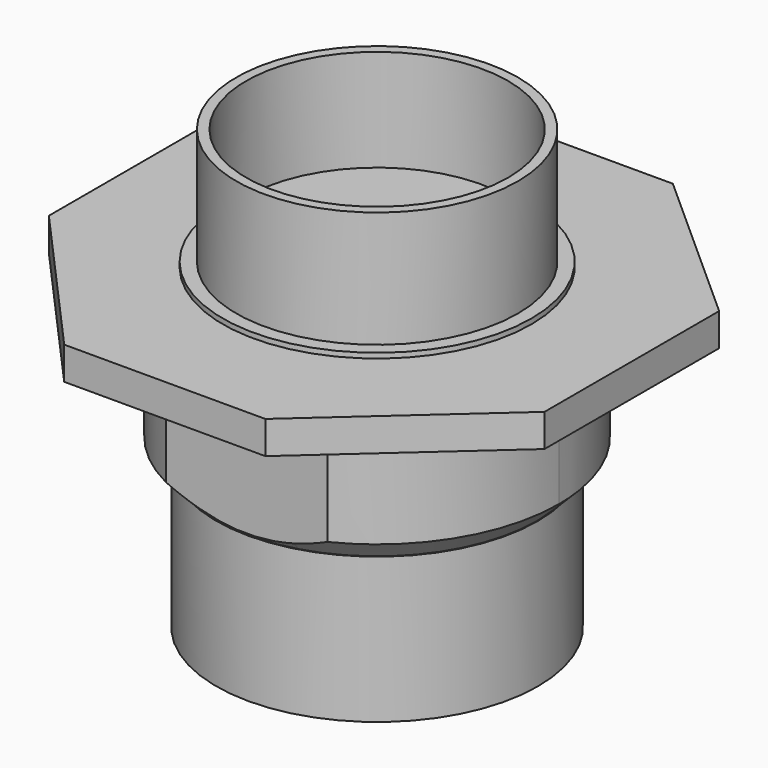
from build123d import *

# Parameters (mm, degrees)
F1_DEPTH    = 2.25
F2_R        = 10.6
F3_DEPTH    = 10.6
F5_DEPTH    = 9.5
F6_T2_ANGLE = 286.1981288485
F6_T4_ANGLE = 106.0815039342
F7_R        = 11.05
F8_DEPTH    = 10
F9_R        = 9
F10_DEPTH   = 7
F11_R       = 10.6
F11_R_2     = 9.6734059383
F12_DEPTH   = 8
F13_R       = 9.375
F14_DEPTH   = 1


# Not quite as in the source:
# - a fillet or chamfer that OpenCascade refuses, or shapes differently, is made with other operations: its cross-section is extruded or revolved along the edge and cut away or added


with BuildPart() as f1:
    # F0 (on Top) → F1 (new body)
    with BuildSketch(Plane.XY):
        Polygon((0, 11.1803398875), (10, 0), (23.8196601125, 0), (35, 10), (35, 25), (23.8196601125, 35), (10, 35), (0, 23.8196601125), align=None)
    extrude(amount=F1_DEPTH)

    # F2 (on Top) → F3 (join)
    with BuildSketch(Plane.XY):
        with Locations((17.5, 17.5)):
            Circle(F2_R)
    extrude(amount=F3_DEPTH)

    # F4 (on face) → F5 (join)
    with BuildSketch(Plane(origin=(0, 0, 0), x_dir=(1, 0, 0), z_dir=(0, 0, -1))):
        with BuildLine():
            ThreePointArc((11.9493243654, -6.3), (10.909607198, -28.1215216761), (30, -17.5))
            ThreePointArc((30, -17.5), (28.1215216761, -10.909607198), (23.0506756346, -6.3))
            Line((23.0506756346, -6.3), (11.9493243654, -6.3))
        make_face()
    extrude(amount=F5_DEPTH)

    # F6: chamfer of 1.5 on 2 edges, made by hand

    # F6_s1 → F6_t2 (revolve, cut)
    with BuildSketch(Plane(origin=(20.8261774668, 6.0498263405, 0), x_dir=(0, 0, 1), z_dir=(0.9603027964, 0.2789597449, 0))):
        with BuildLine():
            Line((-7.9575735931, 0.618923005), (-9.5424264069, -0.9659298087))
            Line((-9.5424264069, -0.9659298087), (-9.5724264069, -0.9659298087))
            ThreePointArc((-9.5724264069, -0.9659298087), (-9.53, -0.1947166053), (-9.53, 0.5764965982))
            Line((-9.53, 0.5764965982), (-9.5, 0.6064965982))
            ThreePointArc((-9.5, 0.6064965982), (-8.7287867966, 0.6064965982), (-7.9575735931, 0.648923005))
            Line((-7.9575735931, 0.648923005), (-7.9575735931, 0.618923005))
        make_face()
    revolve(axis=Axis((17.5, 17.5, -9.5), (0, 0, -1)), revolution_arc=F6_T2_ANGLE, mode=Mode.SUBTRACT)

    # F6_s3 → F6_t4 (revolve, cut)
    with BuildSketch(Plane.XZ.offset(-17.5)):
        with BuildLine():
            Line((30.0424264069, -7.9575735931), (28.4575735931, -9.5424264069))
            Line((28.4575735931, -9.5424264069), (28.4575735931, -9.5724264069))
            ThreePointArc((28.4575735931, -9.5724264069), (29.2287867966, -9.53), (30, -9.53))
            Line((30, -9.53), (30.03, -9.5))
            ThreePointArc((30.03, -9.5), (30.03, -8.7287867966), (30.0724264069, -7.9575735931))
            Line((30.0724264069, -7.9575735931), (30.0424264069, -7.9575735931))
        make_face()
    revolve(axis=Axis((17.5, 17.5, -9.5), (0, 0, -1)), revolution_arc=F6_T4_ANGLE, mode=Mode.SUBTRACT)

    # F7 (on face) → F8 (join)
    with BuildSketch(Plane(origin=(0, 0, -9.5), x_dir=(1, 0, 0), z_dir=(0, 0, -1))):
        with Locations((17.5, -17.5)):
            Circle(F7_R)
    extrude(amount=F8_DEPTH)

    # F9 (on face) → F10 (cut)
    with BuildSketch(Plane.XY.offset(10.6)):
        with Locations((17.5, 17.5)):
            Circle(F9_R)
    extrude(amount=-F10_DEPTH, mode=Mode.SUBTRACT)

    # F11 (on face) → F12 (cut)
    with BuildSketch(Plane.XY.offset(10.6)):
        with Locations((17.5, 17.5)):
            Circle(F11_R)
        with Locations((17.5, 17.5)):
            Circle(F11_R_2, mode=Mode.SUBTRACT)
    extrude(amount=-F12_DEPTH, mode=Mode.SUBTRACT)

    # F13 (on face) → F14 (cut)
    with BuildSketch(Plane(origin=(0, 0, -19.5), x_dir=(1, 0, 0), z_dir=(0, 0, -1))):
        with Locations((17.5, -17.5)):
            Circle(F13_R)
    extrude(amount=-F14_DEPTH, mode=Mode.SUBTRACT)


solid = f1.part
